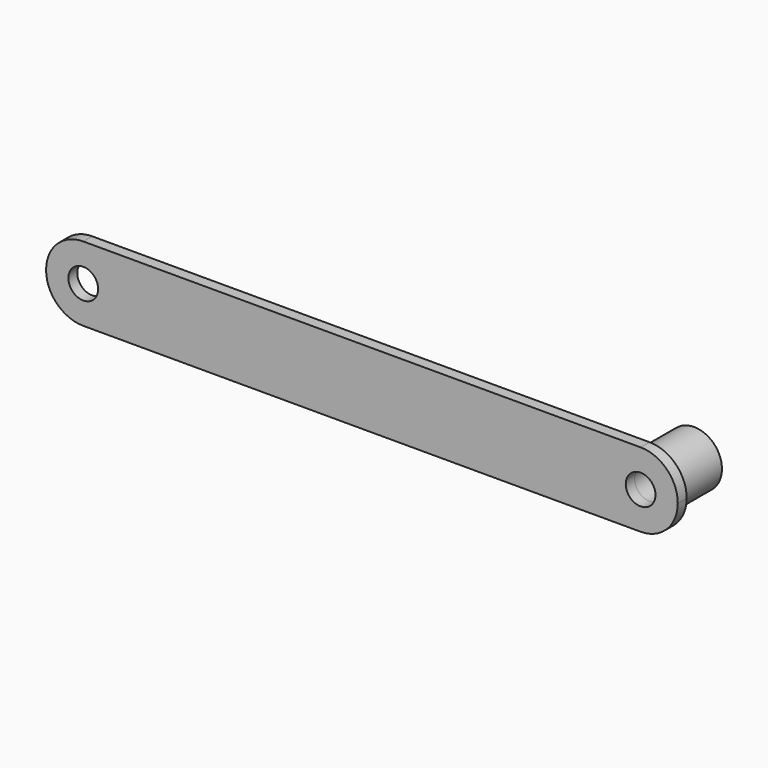
from build123d import *

# Parameters (mm, degrees)
F0_W     = 170
F0_H     = 3
F1_DEPTH = 10
F2_R     = 9.99999
F3_R     = 4
F4_DEPTH = 3
F5_R     = 7.5
F5_R_2   = 4
F6_DEPTH = 15


# Not quite as in the source:
# - a fillet or chamfer is up to 0.001 mm smaller than in the source, because OpenCascade refuses the exact size


with BuildPart() as f1:
    # F0 (on Top) → F1 (new body, symmetric)
    with BuildSketch(Plane.XY):
        Rectangle(F0_W, F0_H)
    extrude(amount=F1_DEPTH, both=True)

    # F2 (radius 10 in the source; OpenCascade refuses exactly that, so slightly less here)
    f2_edges = [f1.edges().sort_by_distance(p)[0] for p in [
        (-85, 0, 10),
        (-85, 0, -10),
        (85, 0, 10),
        (85, 0, -10),
    ]]
    fillet(f2_edges, radius=F2_R)

    # F3 (on face) → F4 (cut, through all)
    with BuildSketch(Plane(origin=(0, 1.5, 0), x_dir=(-1, 0, 0), z_dir=(0, 1, 0))):
        with Locations((-75, 0)):
            Circle(F3_R)
        with Locations((75, 0)):
            Circle(F3_R)
    extrude(amount=-F4_DEPTH, mode=Mode.SUBTRACT)


with BuildPart() as f6:
    # F5 (on face) → F6 (new body)
    with BuildSketch(Plane(origin=(0, 1.5, 0), x_dir=(-1, 0, 0), z_dir=(0, 1, 0))):
        with Locations((-75, 0)):
            Circle(F5_R)
        with Locations((-75, 0)):
            Circle(F5_R_2, mode=Mode.SUBTRACT)
    extrude(amount=F6_DEPTH)


solid = Compound([f1.part, f6.part])
